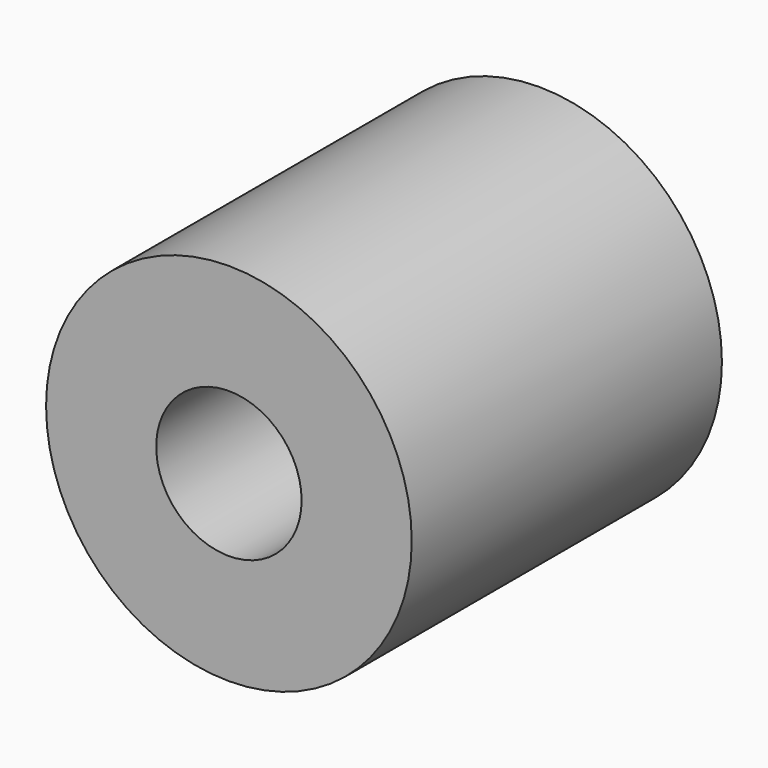
from build123d import *

# Parameters (mm, degrees)
F0_R     = 11.9761
F0_R_2   = 4.7625
F1_DEPTH = 25.4


# Not quite as in the source:
# - a feature names something its author has since deleted; it is built from what else it names


with BuildPart() as f1:
    # F0 (on Front) → F1 (new body)
    with BuildSketch(Plane.XZ):
        Circle(F0_R)
        Circle(F0_R_2, mode=Mode.SUBTRACT)
    extrude(amount=F1_DEPTH)


solid = f1.part
